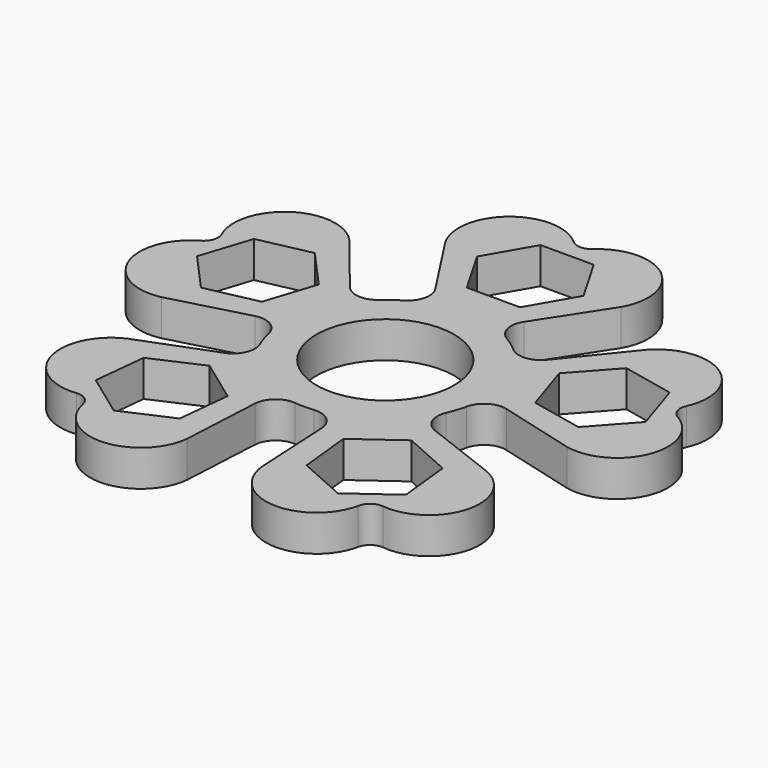
from build123d import *

# Parameters (mm, degrees)
F0_R     = 9.5
F1_DEPTH = 5


# Not quite as in the source:
# - a feature names something its author has since deleted; it is built from what else it names


with BuildPart() as f1:
    # F0 (on Top) → F1 (new body)
    with BuildSketch(Plane.XY):
        with BuildLine():
            ThreePointArc((-13.665469042, -3.0319204432), (-13.3159762762, 4.3418317), (-9.2645390994, 10.5127491897))
            ThreePointArc((-9.2645390994, 10.5127491897), (-11.4998669549, 9.7726015122), (-13.5809814233, 10.8741784618))
            Line((-13.5809814233, 10.8741784618), (-20.506494271, 19.426474585))
            ThreePointArc((-20.506494271, 19.426474585), (-29.538567909, 20.601795911), (-32.0861364699, 11.8571044442))
            ThreePointArc((-32.0861364699, 11.8571044442), (-32.0062029861, 10.4146544851), (-32.9187213461, 9.2946716776))
            ThreePointArc((-32.9187213461, 9.2946716776), (-35.997695766, 0.7226444411), (-27.9997581563, -3.6354203143))
            Line((-27.9997581563, -3.6354203143), (-17.3699870332, -0.7871817262))
            ThreePointArc((-17.3699870332, -0.7871817262), (-15.0388393758, -1.1192356462), (-13.665469042, -3.0319204432))
        make_face()
        Polygon((-28.6916231536, 13.1985965214), (-21.5082094645, 14.7254782362), (-16.5941842664, 9.267900353), (-18.8635727573, 2.2834407549), (-26.0469864464, 0.7565590401), (-30.9610116446, 6.2141369233), align=None, mode=Mode.SUBTRACT)
        with BuildLine():
            ThreePointArc((9.2621690031, 10.5127491897), (8.227808484, 11.3418317), (7.1196691813, 12.0693664265))
            ThreePointArc((7.1196691813, 12.0693664265), (-0.0011850481, 14.0155937788), (-7.1220392775, 12.0693664265))
            ThreePointArc((-7.1220392775, 12.0693664265), (-8.2301785802, 11.3418317), (-9.2645390994, 10.5127491897))
            ThreePointArc((-9.2645390994, 10.5127491897), (-13.3159762762, 4.3418317), (-13.665469042, -3.0319204432))
            ThreePointArc((-13.665469042, -3.0319204432), (-13.3159762762, -4.3106441425), (-12.847106931, -5.5505800398))
            ThreePointArc((-12.847106931, -5.5505800398), (-8.2301785802, -11.3106441425), (-1.3253227589, -13.9216462393))
            ThreePointArc((-1.3253227589, -13.9216462393), (-0.0011850481, -13.9844062212), (1.3229526627, -13.9216462393))
            ThreePointArc((1.3229526627, -13.9216462393), (8.227808484, -11.3106441425), (12.8447368348, -5.5505800398))
            ThreePointArc((12.8447368348, -5.5505800398), (13.31360618, -4.3106441425), (13.6630989458, -3.0319204432))
            ThreePointArc((13.6630989458, -3.0319204432), (13.9146328566, -1.5173811207), (13.9988149519, 0.0155937788))
            ThreePointArc((13.9988149519, 0.0155937788), (12.7598289539, 5.7737637694), (9.2621690031, 10.5127491897))
        make_face()
        Circle(F0_R, mode=Mode.SUBTRACT)
        with BuildLine():
            ThreePointArc((-1.3253227589, -13.9216462393), (-8.2301785802, -11.3106441425), (-12.847106931, -5.5505800398))
            ThreePointArc((-12.847106931, -5.5505800398), (-12.8339389546, -7.9052213736), (-14.5247006287, -9.5440728519))
            Line((-14.5247006287, -9.5440728519), (-24.7985187507, -13.4878221314))
            ThreePointArc((-24.7985187507, -13.4878221314), (-28.7073800051, -21.7146403569), (-21.1779261823, -26.8397803113))
            ThreePointArc((-21.1779261823, -26.8397803113), (-19.7813739443, -27.2095006015), (-18.998190678, -28.4234508549))
            ThreePointArc((-18.998190678, -28.4234508549), (-11.7971637379, -34.0006316328), (-5.1808992125, -27.7408570242))
            Line((-5.1808992125, -27.7408570242), (-4.6049551583, -16.7511898031))
            ThreePointArc((-4.6049551583, -16.7511898031), (-3.5687888714, -14.6367469374), (-1.3253227589, -13.9216462393))
        make_face()
        Polygon((-21.4047986615, -23.1968624525), (-20.6371525584, -15.8931976559), (-13.9281702523, -12.906166284), (-7.9868340493, -17.2227997087), (-8.7544801524, -24.5264645053), (-15.4634624585, -27.5134958771), align=None, mode=Mode.SUBTRACT)
        with BuildLine():
            ThreePointArc((7.1196691813, 12.0693664265), (5.7249926142, 13.9665713389), (6.1295548123, 16.2862348132))
            Line((6.1295548123, 16.2862348132), (12.1231706049, 25.5155937788))
            ThreePointArc((12.1231706049, 25.5155937788), (10.4499033622, 34.4688005315), (1.34596558, 34.1894239382))
            ThreePointArc((1.34596558, 34.1894239382), (-0.0011850481, 33.6676611266), (-1.3483356762, 34.1894239382))
            ThreePointArc((-1.3483356762, 34.1894239382), (-10.4522734584, 34.4688005315), (-12.1255407011, 25.5155937788))
            Line((-12.1255407011, 25.5155937788), (-6.1319249085, 16.2862348132))
            ThreePointArc((-6.1319249085, 16.2862348132), (-5.7273627104, 13.9665713389), (-7.1220392775, 12.0693664265))
            ThreePointArc((-7.1220392775, 12.0693664265), (-0.0011850481, 14.0155937788), (7.1196691813, 12.0693664265))
        make_face()
        Polygon((-7.3450804722, 25.0155937788), (-3.6731327602, 31.3755937788), (3.6707626639, 31.3755937788), (7.342710376, 25.0155937788), (3.6707626639, 18.6555937788), (-3.6731327602, 18.6555937788), align=None, mode=Mode.SUBTRACT)
        with BuildLine():
            ThreePointArc((14.5223305325, -9.5440728519), (12.8315688584, -7.9052213736), (12.8447368348, -5.5505800398))
            ThreePointArc((12.8447368348, -5.5505800398), (8.227808484, -11.3106441425), (1.3229526627, -13.9216462393))
            ThreePointArc((1.3229526627, -13.9216462393), (3.5664187752, -14.6367469374), (4.6025850621, -16.7511898031))
            Line((4.6025850621, -16.7511898031), (5.1785291162, -27.7408570242))
            ThreePointArc((5.1785291162, -27.7408570242), (11.7947936417, -34.0006316328), (18.9958205818, -28.4234508549))
            ThreePointArc((18.9958205818, -28.4234508549), (19.7790038481, -27.2095006015), (21.1755560861, -26.8397803113))
            ThreePointArc((21.1755560861, -26.8397803113), (28.7050099089, -21.7146403569), (24.7961486545, -13.4878221314))
            Line((24.7961486545, -13.4878221314), (14.5223305325, -9.5440728519))
        make_face()
        Polygon((7.9844639531, -17.2227997087), (13.9258001561, -12.906166284), (20.6347824622, -15.8931976559), (21.4024285653, -23.1968624525), (15.4610923623, -27.5134958771), (8.7521100562, -24.5264645053), align=None, mode=Mode.SUBTRACT)
        with BuildLine():
            ThreePointArc((13.5786113271, 10.8741784618), (11.4974968587, 9.7726015122), (9.2621690031, 10.5127491897))
            ThreePointArc((9.2621690031, 10.5127491897), (12.7598289539, 5.7737637694), (13.9988149519, 0.0155937788))
            ThreePointArc((13.9988149519, 0.0155937788), (13.9146328566, -1.5173811207), (13.6630989458, -3.0319204432))
            ThreePointArc((13.6630989458, -3.0319204432), (15.0364692796, -1.1192356462), (17.367616937, -0.7871817262))
            Line((17.367616937, -0.7871817262), (27.99738806, -3.6354203143))
            ThreePointArc((27.99738806, -3.6354203143), (35.9953256698, 0.7226444411), (32.9163512498, 9.2946716776))
            ThreePointArc((32.9163512498, 9.2946716776), (32.0038328898, 10.4146544851), (32.0837663737, 11.8571044442))
            ThreePointArc((32.0837663737, 11.8571044442), (29.5361978128, 20.601795911), (20.5041241748, 19.426474585))
            Line((20.5041241748, 19.426474585), (13.5786113271, 10.8741784618))
        make_face()
        Polygon((18.8612026611, 2.2834407549), (16.5918141702, 9.267900353), (21.5058393683, 14.7254782362), (28.6892530574, 13.1985965214), (30.9586415484, 6.2141369233), (26.0446163502, 0.7565590401), align=None, mode=Mode.SUBTRACT)
    extrude(amount=F1_DEPTH)


solid = f1.part
